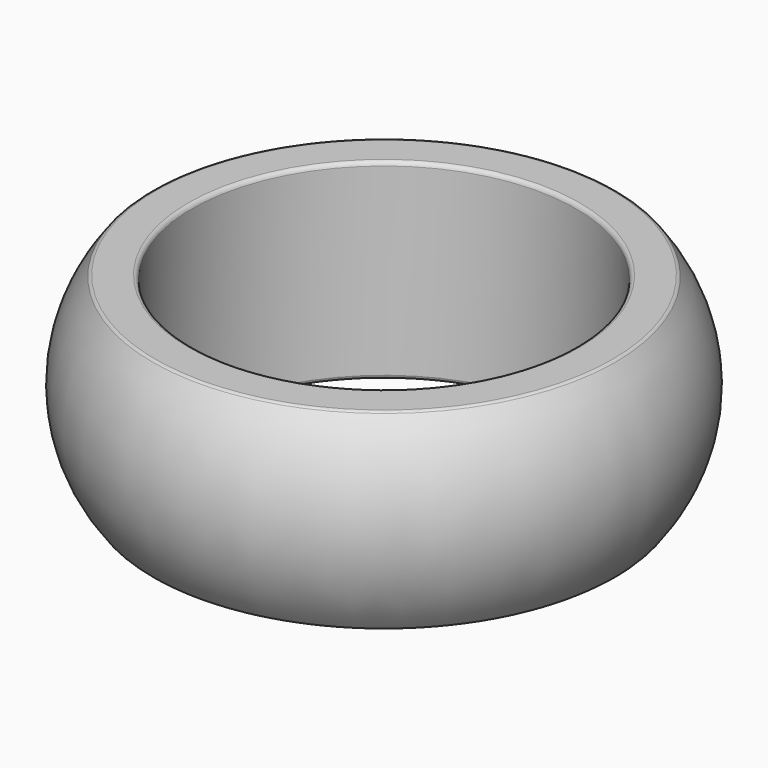
from build123d import *

# Parameters (mm, degrees)
F3_R = 0.1


with BuildPart() as f2:
    # F2: sweep along a path in F0
    with BuildLine(Plane.XY) as f2_path:
        CenterArc((0, 0), 5, 0, 360)
    # F1 (on Front) → F2 (sweep)
    with BuildSketch(Plane.XZ):
        with BuildLine():
            Line((-6, 0), (-5, 0))
            Line((-5, 0), (-5, 5))
            Line((-5, 5), (-6, 5))
            ThreePointArc((-6, 5), (-6.8775010008, 2.5), (-6, 0))
        make_face()
    sweep(path=f2_path.line)

    # F3
    f3_edges = [f2.edges().sort_by_distance(p)[0] for p in [
        (-5, 0, 0),
        (-5, 0, 5),
        (-6, 0, 0),
        (-6, 0, 5),
    ]]
    fillet(f3_edges, radius=F3_R)


solid = f2.part
